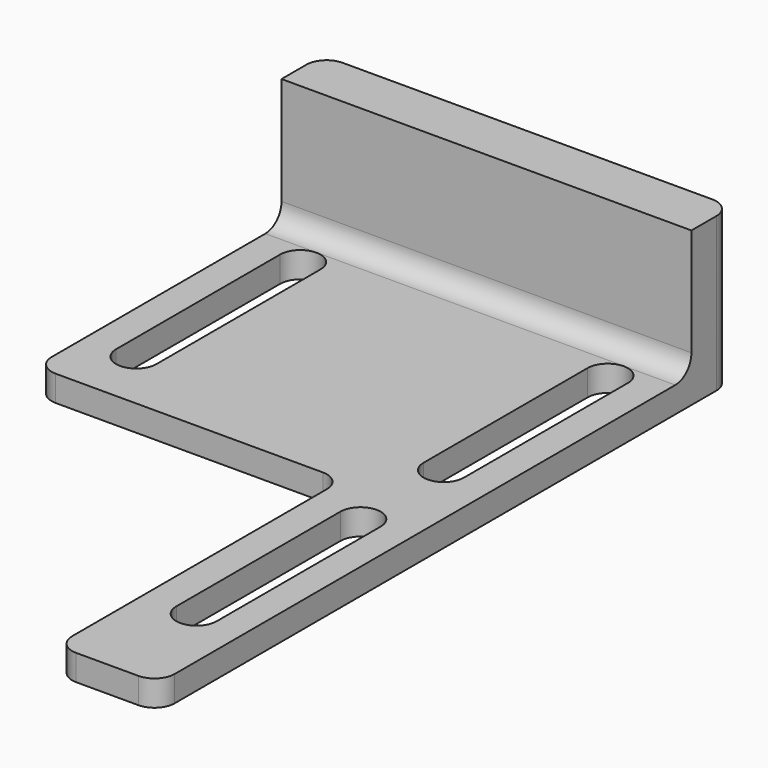
from build123d import *

# Parameters (mm, degrees)
F0_W     = 101.6
F0_H     = 12.7
F1_DEPTH = 6.4
F2_DEPTH = 31.7
F3_DEPTH = 6.4
F4_R     = 5


with BuildPart() as f1:
    # F0 (on Top) → F1 (new body)
    with BuildSketch(Plane.XY):
        Polygon((25.4, -88.9), (50.8, -88.9), (50.8, -10.7497644231), (50.8, 76.2), (-50.8, 76.2), (-50.8, 0), (25.4, 0), align=None)
        with BuildLine():
            ThreePointArc((33.3328473049, -10.7497644231), (38.3328473049, -5.7497644231), (43.3328473049, -10.7497644231))
            Line((43.3328473049, -10.7497644231), (43.3328473049, -61.5497644231))
            ThreePointArc((43.3328473049, -61.5497644231), (38.3328473049, -66.5497644231), (33.3328473049, -61.5497644231))
            Line((33.3328473049, -61.5497644231), (33.3328473049, -10.7497644231))
        make_face(mode=Mode.SUBTRACT)
        with BuildLine():
            Line((-33.0996350241, 66.1321754187), (-33.0996350241, 15.3321754187))
            ThreePointArc((-33.0996350241, 15.3321754187), (-38.0996350241, 10.3321754187), (-43.0996350241, 15.3321754187))
            Line((-43.0996350241, 15.3321754187), (-43.0996350241, 66.1321754187))
            ThreePointArc((-43.0996350241, 66.1321754187), (-38.0996350241, 71.1321754187), (-33.0996350241, 66.1321754187))
        make_face(mode=Mode.SUBTRACT)
        with BuildLine():
            Line((43.1003649759, 66.1321754187), (43.1003649759, 15.3321754187))
            ThreePointArc((43.1003649759, 15.3321754187), (38.1003649759, 10.3321754187), (33.1003649759, 15.3321754187))
            Line((33.1003649759, 15.3321754187), (33.1003649759, 66.1321754187))
            ThreePointArc((33.1003649759, 66.1321754187), (38.1003649759, 71.1321754187), (43.1003649759, 66.1321754187))
        make_face(mode=Mode.SUBTRACT)
        Polygon((-25.4, -88.9), (25.4, -88.9), (25.4, 0), (-50.8, 0), (-50.8, -10.0678245813), (-50.8, -88.9), align=None)
        with BuildLine():
            Line((-43.0996350241, -60.8678127293), (-43.0996350241, -10.0678245813))
            ThreePointArc((-43.0996350241, -10.0678245813), (-38.0822904681, -5.0678546647), (-33.0997553575, -10.1025134845))
            Line((-33.0997553575, -10.1025134845), (-33.0996350241, -60.8678127293))
            ThreePointArc((-33.0996350241, -60.8678127293), (-38.0996350241, -65.8678127293), (-43.0996350241, -60.8678127293))
        make_face(mode=Mode.SUBTRACT)
        with Locations((0, 82.55)):
            Rectangle(F0_W, F0_H)
    extrude(amount=-F1_DEPTH)

    # F0 (on Top) → F2 (join)
    with BuildSketch(Plane.XY):
        with Locations((0, 82.55)):
            Rectangle(F0_W, F0_H)
    extrude(amount=F2_DEPTH)

    # F0 (on Top) → F3 (cut)
    with BuildSketch(Plane.XY):
        Polygon((-25.4, -88.9), (25.4, -88.9), (25.4, 0), (-50.8, 0), (-50.8, -10.0678245813), (-50.8, -88.9), align=None)
        with BuildLine():
            Line((-43.0996350241, -60.8678127293), (-43.0996350241, -10.0678245813))
            ThreePointArc((-43.0996350241, -10.0678245813), (-38.0822904681, -5.0678546647), (-33.0997553575, -10.1025134845))
            Line((-33.0997553575, -10.1025134845), (-33.0996350241, -60.8678127293))
            ThreePointArc((-33.0996350241, -60.8678127293), (-38.0996350241, -65.8678127293), (-43.0996350241, -60.8678127293))
        make_face(mode=Mode.SUBTRACT)
    extrude(amount=-F3_DEPTH, mode=Mode.SUBTRACT)

    # F4
    f4_edges = [f1.edges().sort_by_distance(p)[0] for p in [
        (0, 76.2, 0),
        (50.8, 88.9, 12.65),
        (-50.8, 88.9, 12.65),
        (25.4, -88.9, -3.2),
        (50.8, -88.9, -3.2),
        (25.4, 0, -3.2),
        (-50.8, 0, -3.2),
    ]]
    fillet(f4_edges, radius=F4_R)


solid = f1.part
